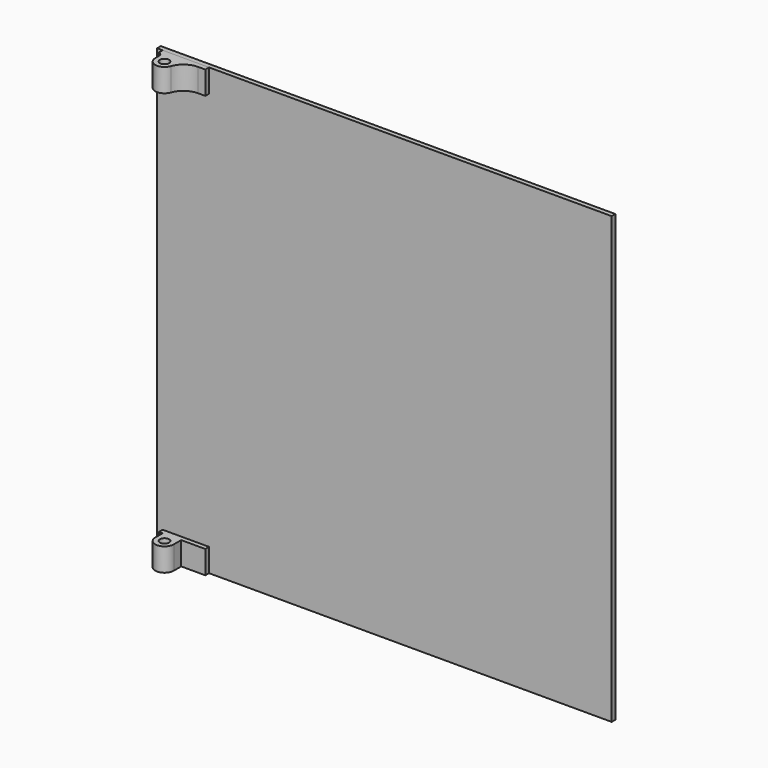
from build123d import *

# Parameters (mm, degrees)
F0_W        = 490
F0_H        = 480
F1_DEPTH    = 5
F2_R        = 5
F3_DEPTH    = 25
F6_R        = 20
F7_T1_DEPTH = 25


# Not quite as in the source:
# - a fillet or chamfer that OpenCascade refuses, or shapes differently, is made with other operations: its cross-section is extruded or revolved along the edge and cut away or added


with BuildPart() as f1:
    # F0 (on Front) → F1 (new body)
    with BuildSketch(Plane.XZ):
        Rectangle(F0_W, F0_H)
    extrude(amount=F1_DEPTH)


with BuildPart() as f3:
    # F2 (on face) → F3 (new body)
    with BuildSketch(Plane.XY.offset(240)):
        Polygon((-189, -10), (-189, -5), (-239, -5), (-239, -10), (-235, -10), (-225, -10), (-215, -10), align=None)
        with BuildLine():
            ThreePointArc((-215, -20), (-217.9289321881, -12.9289321881), (-225, -10))
            ThreePointArc((-225, -10), (-232.0710678119, -12.9289321881), (-235, -20))
            ThreePointArc((-235, -20), (-225, -30), (-215, -20))
        make_face()
        with Locations((-225, -20)):
            Circle(F2_R, mode=Mode.SUBTRACT)
        with BuildLine():
            Line((-215, -20), (-215, -10))
            Line((-215, -10), (-225, -10))
            ThreePointArc((-225, -10), (-217.9289321881, -12.9289321881), (-215, -20))
        make_face()
        with BuildLine():
            Line((-225, -10), (-235, -10))
            Line((-235, -10), (-235, -20))
            ThreePointArc((-235, -20), (-232.0710678119, -12.9289321881), (-225, -10))
        make_face()
    extrude(amount=-F3_DEPTH)


with BuildPart() as f4_1:
    # F4: instance of F3
    add(f3.part.mirror(Plane.XY))


with BuildPart() as f3_1:
    add(f3.part)

    # F6
    f6_edges = [f3_1.edges().sort_by_distance(p)[0] for p in [
        (-215, -10, 227.5),
    ]]
    fillet(f6_edges, radius=F6_R)

    # F7: fillet of radius 5 on 1 edges, made by hand

    # F7_s2 → F7_t1 (join)
    with BuildSketch(Plane.XY.offset(215)):
        with BuildLine():
            ThreePointArc((-235, -14.8989794856), (-236.1270166538, -11.7367018254), (-239, -10))
            Line((-239, -10), (-235, -10))
            Line((-235, -10), (-235, -14.8989794856))
        make_face()
    extrude(amount=F7_T1_DEPTH)


solid = Compound([f1.part, f4_1.part, f3_1.part])
